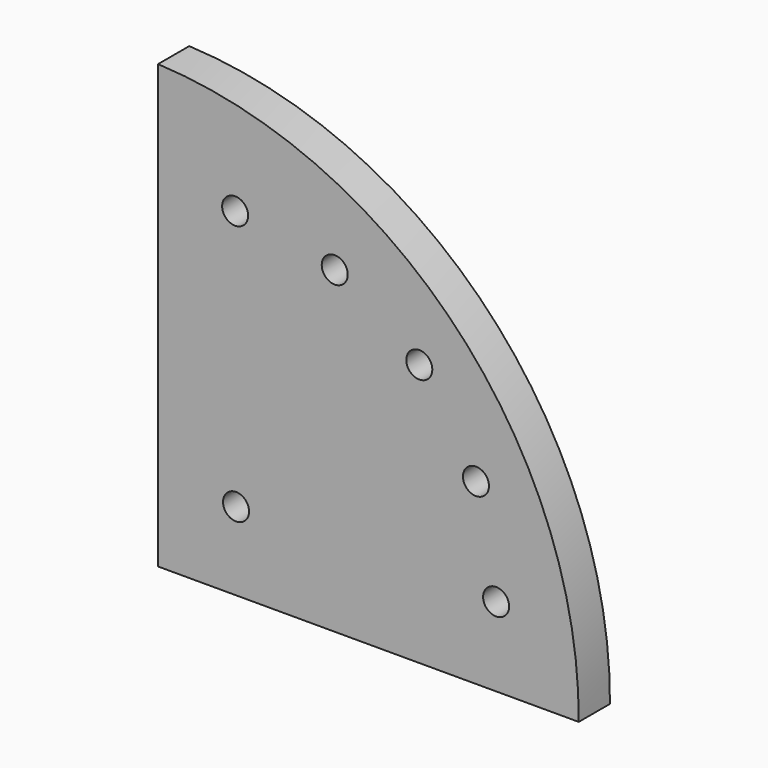
from build123d import *

# Parameters (mm, degrees)
F1_DEPTH = 4.7625
F3_D     = 6.35
F4_R     = 3.175
F5_DEPTH = 25.4


with BuildPart() as f1:
    # F0 (on Front) → F1 (new body, symmetric)
    with BuildSketch(Plane.XZ):
        with BuildLine():
            ThreePointArc((107.4907893633, -0.6147240541), (0, 107.4925471073), (-107.4907893633, -0.6147240541))
            Line((-107.4907893633, -0.6147240541), (107.4907893633, -0.6147240541))
        make_face()
    extrude(amount=F1_DEPTH, both=True)

    # F3 (through all)
    with Locations(Plane.XZ.offset(4.7625)):
        with Locations((23.8125, 18.4352759459), (87.3125, 18.6611738243), (47.9041955289, 77.1880736359), (23.5866021216, 81.9352759459), (68.5540466837, 63.4962904729), (82.392402939, 42.9443763274), (-23.8125, 18.4352759459), (-23.5866021216, 81.9352759459), (-47.9041955289, 77.1880736359), (-68.5540466837, 63.4962904729), (-82.392402939, 42.9443763274), (-87.3125, 18.6611738243)):
            Hole(F3_D / 2)

    # F4 (on face) → F5 (cut)
    with BuildSketch(Plane.XZ.offset(4.7625)):
        with BuildLine():
            Line((-135.8842252305, -8.5859880761), (4.7625, -8.5859880761))
            Line((4.7625, -8.5859880761), (4.7625, -0.6147240541))
            Line((4.7625, -0.6147240541), (-107.4907893633, -0.6147240541))
            ThreePointArc((-107.4907893633, -0.6147240541), (-74.5276330195, 77.4614717141), (4.7625, 107.3869930548))
            Line((4.7625, 107.3869930548), (4.7625, 118.4140119239))
            Line((4.7625, 118.4140119239), (-135.8842252305, 118.4140119239))
            Line((-135.8842252305, 118.4140119239), (-135.8842252305, -8.5859880761))
        make_face()
        with BuildLine():
            Line((-107.4907893633, -0.6147240541), (4.7625, -0.6147240541))
            Line((4.7625, -0.6147240541), (4.7625, 107.3869930548))
            ThreePointArc((4.7625, 107.3869930548), (-74.5276330195, 77.4614717141), (-107.4907893633, -0.6147240541))
        make_face()
        with Locations((-87.3125, 18.6611738243)):
            Circle(F4_R, mode=Mode.SUBTRACT)
        with Locations((-23.8125, 18.4352759459)):
            Circle(F4_R, mode=Mode.SUBTRACT)
        with Locations((-82.392402939, 42.9443763274)):
            Circle(F4_R, mode=Mode.SUBTRACT)
        with Locations((-68.5540466837, 63.4962904729)):
            Circle(F4_R, mode=Mode.SUBTRACT)
        with Locations((-47.9041955289, 77.1880736359)):
            Circle(F4_R, mode=Mode.SUBTRACT)
        with Locations((-23.5866021216, 81.9352759459)):
            Circle(F4_R, mode=Mode.SUBTRACT)
    extrude(amount=-F5_DEPTH, mode=Mode.SUBTRACT)


solid = f1.part
